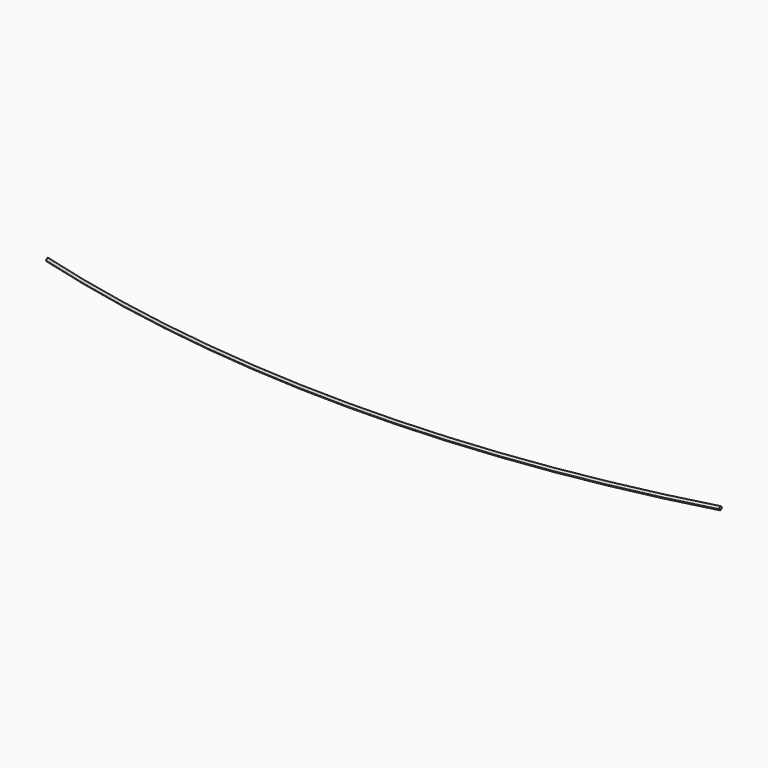
from build123d import *

# Parameters (mm, degrees)
F1_DEPTH    = 5
F2_T2_ANGLE = 31.9892462311
F2_T4_ANGLE = 32.125738606
F2_T6_ANGLE = 31.9892462311
F2_T8_ANGLE = 32.125738606


# Not quite as in the source:
# - a fillet or chamfer that OpenCascade refuses, or shapes differently, is made with other operations: its cross-section is extruded or revolved along the edge and cut away or added


with BuildPart() as f1:
    # F0 (on Top) → F1 (new body)
    with BuildSketch(Plane.XY):
        with BuildLine():
            ThreePointArc((340.9691074047, 0), (20.9691074047, -43.4534164159), (-299.0308925953, 0))
            Line((-299.0308925953, 0), (-299.0308925953, -5.187034764))
            ThreePointArc((-299.0308925953, -5.187034764), (20.9691074047, -48.4534164159), (340.9691074047, -5.187034764))
            Line((340.9691074047, -5.187034764), (340.9691074047, 0))
        make_face()
    extrude(amount=F1_DEPTH)

    # F2: fillet of radius 5 on 4 edges, made by hand

    # F2_s1 → F2_t2 (revolve, cut)
    with BuildSketch(Plane(origin=(-286.9691065764, 82.2579232266, 0), x_dir=(0, 0, 1), z_dir=(-0.9612875587, 0.2755471456, 0))):
        with BuildLine():
            ThreePointArc((5, -87.4481804397), (1.4644660941, -85.9837143456), (0, -82.4481804397))
            Line((0, -82.4481804397), (0, -87.4481804397))
            Line((0, -87.4481804397), (5, -87.4481804397))
        make_face()
    revolve(axis=Axis((20.9691074047, 1156.5465835841, 0), (0, 0, 1)), revolution_arc=F2_T2_ANGLE, mode=Mode.SUBTRACT)

    # F2_s3 → F2_t4 (revolve, cut)
    with BuildSketch(Plane(origin=(326.8773802338, 94.1188689208, 0), x_dir=(0, 0, 1), z_dir=(0.960958667, 0.2766919594, 0))):
        with BuildLine():
            ThreePointArc((0, 94.4085201712), (3.5355339059, 95.8729862653), (5, 99.4085201712))
            Line((5, 99.4085201712), (5, 94.4085201712))
            Line((5, 94.4085201712), (0, 94.4085201712))
        make_face()
    revolve(axis=Axis((20.9691074047, 1156.5465835841, 5), (0, 0, -1)), revolution_arc=F2_T4_ANGLE, mode=Mode.SUBTRACT)

    # F2_s5 → F2_t6 (revolve, cut)
    with BuildSketch(Plane(origin=(-286.9691065764, 82.2579232266, 0), x_dir=(0, 0, 1), z_dir=(-0.9612875587, 0.2755471456, 0))):
        with BuildLine():
            ThreePointArc((0, -87.4481804397), (3.5355339059, -85.9837143456), (5, -82.4481804397))
            Line((5, -82.4481804397), (5, -87.4481804397))
            Line((5, -87.4481804397), (0, -87.4481804397))
        make_face()
    revolve(axis=Axis((20.9691074047, 1156.5465835841, 5), (0, 0, 1)), revolution_arc=F2_T6_ANGLE, mode=Mode.SUBTRACT)

    # F2_s7 → F2_t8 (revolve, cut)
    with BuildSketch(Plane(origin=(326.8773802338, 94.1188689208, 0), x_dir=(0, 0, 1), z_dir=(0.960958667, 0.2766919594, 0))):
        with BuildLine():
            ThreePointArc((5, 94.4085201712), (1.4644660941, 95.8729862653), (0, 99.4085201712))
            Line((0, 99.4085201712), (0, 94.4085201712))
            Line((0, 94.4085201712), (5, 94.4085201712))
        make_face()
    revolve(axis=Axis((20.9691074047, 1156.5465835841, 0), (0, 0, -1)), revolution_arc=F2_T8_ANGLE, mode=Mode.SUBTRACT)


solid = f1.part
